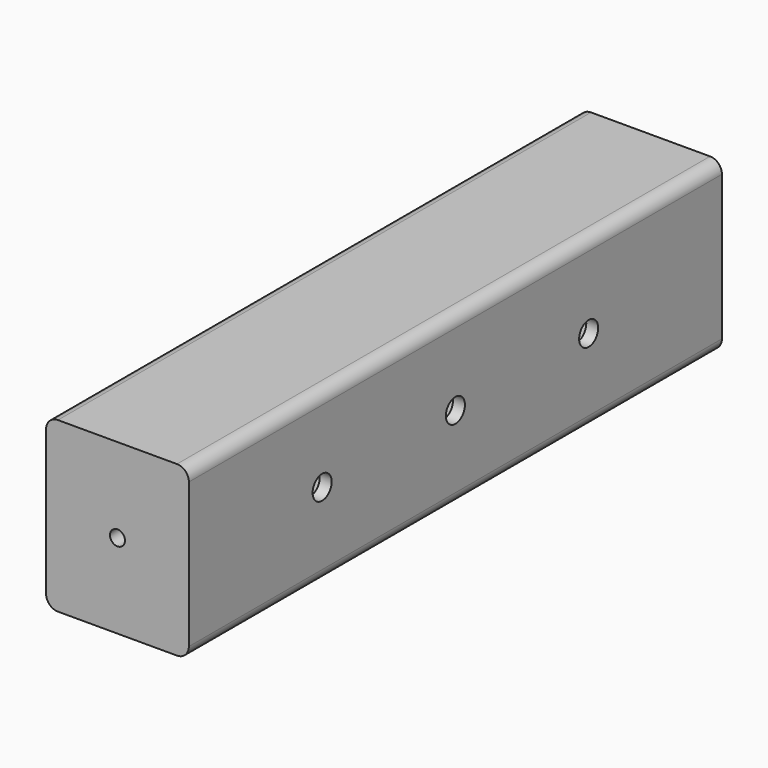
from build123d import *

# Parameters (mm, degrees)
F0_R     = 4
F1_DEPTH = 6.35
F2_DEPTH = 355.6
F4_DEPTH = 12.7
F5_R     = 6.35
F6_DEPTH = 76.201


# Not quite as in the source:
# - a feature names something its author has since deleted; it is built from what else it names


with BuildPart() as f1:
    # F0 (on Front) → F1 (new body)
    with BuildSketch(Plane.XZ):
        with BuildLine():
            Line((-25.4, -38.65), (25.4, -38.65))
            ThreePointArc((25.4, -38.65), (29.8901280605, -36.7901280605), (31.75, -32.3))
            Line((31.75, -32.3), (31.75, 32.3))
            ThreePointArc((31.75, 32.3), (29.8901280605, 36.7901280605), (25.4, 38.65))
            Line((25.4, 38.65), (-25.4, 38.65))
            ThreePointArc((-25.4, 38.65), (-29.8901280605, 36.7901280605), (-31.75, 32.3))
            Line((-31.75, 32.3), (-31.75, -32.3))
            ThreePointArc((-31.75, -32.3), (-29.8901280605, -36.7901280605), (-25.4, -38.65))
        make_face()
        Circle(F0_R, mode=Mode.SUBTRACT)
    extrude(amount=-F1_DEPTH)

    # F0 (on Front) → F2 (join)
    with BuildSketch(Plane.XZ):
        with BuildLine():
            Line((-31.75, -45), (31.75, -45))
            ThreePointArc((31.75, -45), (36.2401280605, -43.1401280605), (38.1, -38.65))
            Line((38.1, -38.65), (38.1, 38.65))
            ThreePointArc((38.1, 38.65), (36.2401280605, 43.1401280605), (31.75, 45))
            Line((31.75, 45), (-31.75, 45))
            ThreePointArc((-31.75, 45), (-36.2401280605, 43.1401280605), (-38.1, 38.65))
            Line((-38.1, 38.65), (-38.1, -38.65))
            ThreePointArc((-38.1, -38.65), (-36.2401280605, -43.1401280605), (-31.75, -45))
        make_face()
        with BuildLine():
            ThreePointArc((31.75, -32.3), (29.8901280605, -36.7901280605), (25.4, -38.65))
            Line((25.4, -38.65), (-25.4, -38.65))
            ThreePointArc((-25.4, -38.65), (-29.8901280605, -36.7901280605), (-31.75, -32.3))
            Line((-31.75, -32.3), (-31.75, 32.3))
            ThreePointArc((-31.75, 32.3), (-29.8901280605, 36.7901280605), (-25.4, 38.65))
            Line((-25.4, 38.65), (25.4, 38.65))
            ThreePointArc((25.4, 38.65), (29.8901280605, 36.7901280605), (31.75, 32.3))
            Line((31.75, 32.3), (31.75, -32.3))
        make_face(mode=Mode.SUBTRACT)
    extrude(amount=-F2_DEPTH)

    # F0 (on Front) → F4 (join)
    with BuildSketch(Plane.XZ):
        with BuildLine():
            Line((-31.75, -45), (31.75, -45))
            ThreePointArc((31.75, -45), (36.2401280605, -43.1401280605), (38.1, -38.65))
            Line((38.1, -38.65), (38.1, 38.65))
            ThreePointArc((38.1, 38.65), (36.2401280605, 43.1401280605), (31.75, 45))
            Line((31.75, 45), (-31.75, 45))
            ThreePointArc((-31.75, 45), (-36.2401280605, 43.1401280605), (-38.1, 38.65))
            Line((-38.1, 38.65), (-38.1, -38.65))
            ThreePointArc((-38.1, -38.65), (-36.2401280605, -43.1401280605), (-31.75, -45))
        make_face()
        with BuildLine():
            ThreePointArc((31.75, -32.3), (29.8901280605, -36.7901280605), (25.4, -38.65))
            Line((25.4, -38.65), (-25.4, -38.65))
            ThreePointArc((-25.4, -38.65), (-29.8901280605, -36.7901280605), (-31.75, -32.3))
            Line((-31.75, -32.3), (-31.75, 32.3))
            ThreePointArc((-31.75, 32.3), (-29.8901280605, 36.7901280605), (-25.4, 38.65))
            Line((-25.4, 38.65), (25.4, 38.65))
            ThreePointArc((25.4, 38.65), (29.8901280605, 36.7901280605), (31.75, 32.3))
            Line((31.75, 32.3), (31.75, -32.3))
        make_face(mode=Mode.SUBTRACT)
        with BuildLine():
            Line((-25.4, -38.65), (25.4, -38.65))
            ThreePointArc((25.4, -38.65), (29.8901280605, -36.7901280605), (31.75, -32.3))
            Line((31.75, -32.3), (31.75, 32.3))
            ThreePointArc((31.75, 32.3), (29.8901280605, 36.7901280605), (25.4, 38.65))
            Line((25.4, 38.65), (-25.4, 38.65))
            ThreePointArc((-25.4, 38.65), (-29.8901280605, 36.7901280605), (-31.75, 32.3))
            Line((-31.75, 32.3), (-31.75, -32.3))
            ThreePointArc((-31.75, -32.3), (-29.8901280605, -36.7901280605), (-25.4, -38.65))
        make_face()
        Circle(F0_R, mode=Mode.SUBTRACT)
    extrude(amount=-F4_DEPTH)

    # F5 (on face) → F6 (cut, through all)
    with BuildSketch(Plane.YZ.offset(38.1)):
        with Locations((88.9, 0)):
            Circle(F5_R)
        with Locations((177.8, 0)):
            Circle(F5_R)
        with Locations((266.7, 0)):
            Circle(F5_R)
    extrude(amount=-F6_DEPTH, mode=Mode.SUBTRACT)


solid = f1.part
